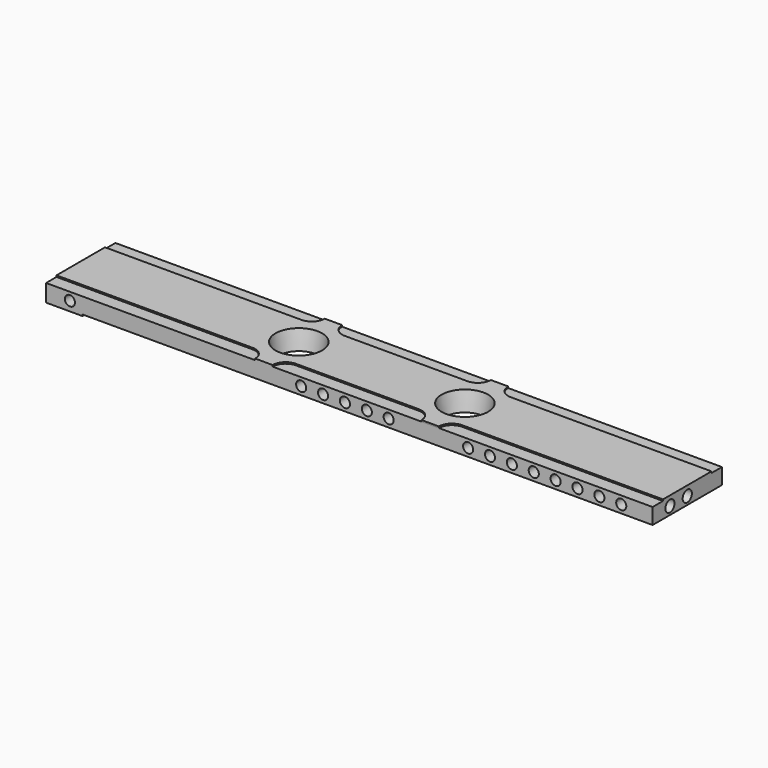
from build123d import *

# Parameters (mm, degrees)
F1_DEPTH  = 13
F2_R      = 16.11
F3_DEPTH  = 16
F3_TAPER  = 8.7
F5_DEPTH  = 1
F6_R      = 3.5
F7_DEPTH  = 60
F9_DEPTH  = 1
F10_DEPTH = 1
F11_DEPTH = 1
F12_DEPTH = 1
F13_R     = 2.625
F14_DEPTH = 15
F15_R     = 3.975
F16_DEPTH = 12.36


# Not quite as in the source:
# - ends of sketch curves that miss each other by under 0.0002 mm in the source are joined


with BuildPart() as f1:
    # F0 (on Top) → F1 (new body)
    with BuildSketch(Plane.XY):
        Polygon((-210, -30), (210, -30), (210, 30), (-210, 30), (-210, 21), (-210, -21), align=None)
    extrude(amount=F1_DEPTH)

    # F2 (on face) → F3 (cut)
    with BuildSketch(Plane.XY.offset(13)):
        with Locations((56, 0)):
            Circle(F2_R)
        with Locations((-59, 0)):
            Circle(F2_R)
    extrude(amount=-F3_DEPTH, taper=F3_TAPER, mode=Mode.SUBTRACT)

    # F4 (on face) → F5 (cut)
    with BuildSketch(Plane(origin=(0, 0, 0), x_dir=(1, 0, 0), z_dir=(0, 0, -1))):
        with BuildLine():
            Line((210, 30), (-184.9498743711, 30))
            ThreePointArc((-184.9498743711, 30), (-181.7082039325, 23.5838015129), (-175, 21))
            Line((-175, 21), (150, 21))
            ThreePointArc((150, 21), (171, 0), (150, -21))
            Line((150, -21), (-175, -21))
            ThreePointArc((-175, -21), (-181.7082039325, -23.5838015129), (-184.9498743711, -30))
            Line((-184.9498743711, -30), (210, -30))
            Line((210, -30), (210, 30))
        make_face()
    extrude(amount=-F5_DEPTH, mode=Mode.SUBTRACT)

    # F6 (on face) → F7 (cut)
    with BuildSketch(Plane(origin=(0, 30, 0), x_dir=(-1, 0, 0), z_dir=(0, 1, 0))):
        with BuildLine():
            ThreePointArc((190, 6.5), (193.5, 3), (197, 6.5))
            Line((197, 6.5), (193.5, 6.5))
            Line((193.5, 6.5), (190, 6.5))
        make_face()
        with BuildLine():
            Line((193.5, 6.5), (197, 6.5))
            ThreePointArc((197, 6.5), (193.5, 10), (190, 6.5))
            Line((190, 6.5), (193.5, 6.5))
        make_face()
        with Locations((33.35, 6.5)):
            Circle(F6_R)
        with Locations((18.2, 6.5)):
            Circle(F6_R)
        with Locations((3.05, 6.5)):
            Circle(F6_R)
        with Locations((-12.1, 6.5)):
            Circle(F6_R)
        with BuildLine():
            ThreePointArc((-30.75, 6.5), (-27.25, 3), (-23.75, 6.5))
            ThreePointArc((-23.75, 6.5), (-27.25, 10), (-30.75, 6.5))
        make_face()
        with Locations((-82.25, 6.5)):
            Circle(F6_R)
        with Locations((-97.4, 6.5)):
            Circle(F6_R)
        with Locations((-112.55, 6.5)):
            Circle(F6_R)
        with Locations((-127.7, 6.5)):
            Circle(F6_R)
        with Locations((-142.85, 6.5)):
            Circle(F6_R)
        with Locations((-158, 6.5)):
            Circle(F6_R)
        with Locations((-173.15, 6.5)):
            Circle(F6_R)
        with Locations((-188.3, 6.5)):
            Circle(F6_R)
    extrude(amount=-F7_DEPTH, mode=Mode.SUBTRACT)

    # F8 (on face) → F9 (cut)
    with BuildSketch(Plane.XY.offset(13)):
        with BuildLine():
            Line((210, 30), (62, 30))
            ThreePointArc((62, 30), (64.6360389693, 23.6360389693), (71, 21))
            Line((71, 21), (210, 21))
            Line((210, 21), (210, 30))
        make_face()
    extrude(amount=-F9_DEPTH, mode=Mode.SUBTRACT)

    # F8 (on face) → F10 (cut)
    with BuildSketch(Plane.XY.offset(13)):
        with BuildLine():
            Line((210, -30), (210, -21))
            Line((210, -21), (71, -21))
            ThreePointArc((71, -21), (64.6360389693, -23.6360389693), (62, -30))
            Line((62, -30), (210, -30))
        make_face()
        with BuildLine():
            ThreePointArc((-44.1668648796, -21), (-50.5308259103, -23.6360389693), (-53.1668648796, -30))
            Line((-53.1668648796, -30), (50, -30))
            Line((50, -30), (61.9996917391, -30))
            Line((61.9996917391, -30), (61.9996917391, -29.9984586954))
            Line((61.9996917391, -29.9984586954), (49.9996917391, -29.9984586954))
            Line((49.9996917391, -29.9984586954), (49.9966373946, -29.8334433813))
            ThreePointArc((49.9966373946, -29.8334433813), (47.3029780787, -23.5774222633), (40.9981786992, -21))
            Line((40.9981786992, -21), (-44.1668648796, -21))
        make_face()
    extrude(amount=-F10_DEPTH, mode=Mode.SUBTRACT)

    # F8 (on face) → F11 (cut)
    with BuildSketch(Plane.XY.offset(13)):
        with BuildLine():
            Line((-74.1668648796, -21), (-210, -21))
            Line((-210, -21), (-210, -30))
            Line((-210, -30), (-65.1668648796, -30))
            ThreePointArc((-65.1668648796, -30), (-67.8029038489, -23.6360389693), (-74.1668648796, -21))
        make_face()
        with BuildLine():
            ThreePointArc((-73.9996917391, 21), (-67.6362756652, 23.6354940592), (-64.9996918711, 29.9984586954))
            Line((-64.9996918711, 29.9984586954), (-64.9996917391, 30))
            Line((-64.9996917391, 30), (-210, 30))
            Line((-210, 30), (-210, 21))
            Line((-210, 21), (-73.9996917391, 21))
        make_face()
    extrude(amount=-F11_DEPTH, mode=Mode.SUBTRACT)

    # F8 (on face) → F12 (cut)
    with BuildSketch(Plane.XY.offset(13)):
        with BuildLine():
            Line((50, 30), (-52.9996917391, 30))
            Line((-52.9996917391, 30), (-52.9996917391, 29.9969173908))
            ThreePointArc((-52.9996917391, 29.9969173908), (-50.3636527698, 23.6329563601), (-43.9996917391, 20.9969173908))
            Line((-43.9996917391, 20.9969173908), (41.0002951444, 20.9997048653))
            ThreePointArc((41.0002951444, 20.9997048653), (47.3640653791, 23.6358481799), (50, 29.9997048604))
            Line((50, 29.9997048604), (50, 30))
        make_face()
    extrude(amount=-F12_DEPTH, mode=Mode.SUBTRACT)

    # F13 (on face) → F14 (cut)
    with BuildSketch(Plane(origin=(-210, 0, 0), x_dir=(0, -1, 0), z_dir=(-1, 0, 0))):
        with Locations((-20, 8)):
            Circle(F13_R)
        with Locations((20, 8)):
            Circle(F13_R)
    extrude(amount=-F14_DEPTH, mode=Mode.SUBTRACT)

    # F15 (on face) → F16 (cut)
    with BuildSketch(Plane.YZ.offset(210)):
        with Locations((0, 6.5)):
            Circle(F15_R)
        with Locations((-15, 6.5)):
            Circle(F15_R)
    extrude(amount=-F16_DEPTH, mode=Mode.SUBTRACT)


solid = f1.part
